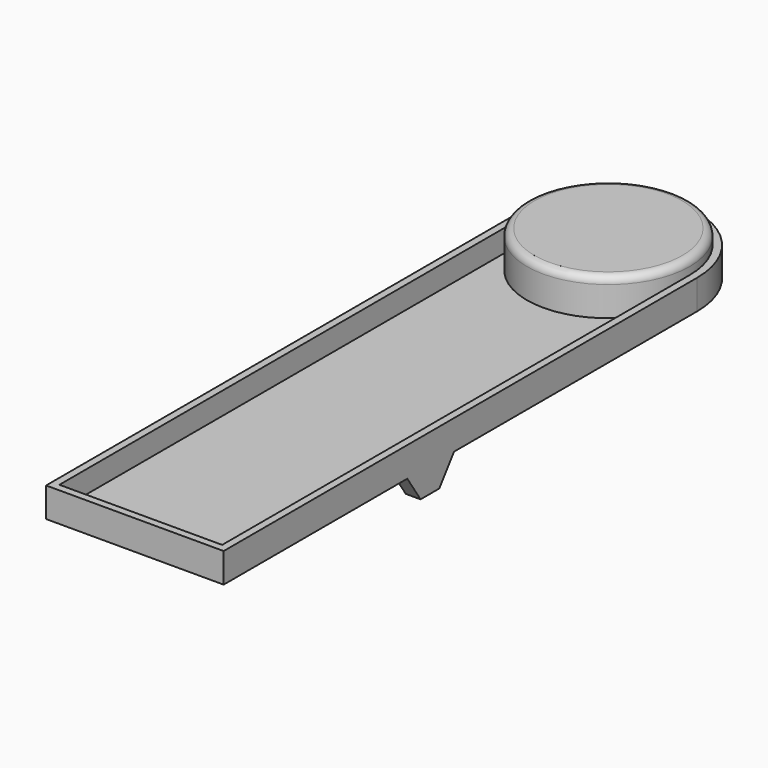
from build123d import *

# Parameters (mm, degrees)
F1_DEPTH = 50.8
F2_T     = -12.7
F3_R     = 139.7
F4_DEPTH = 63.5
F7_DEPTH = 25.4


# Not quite as in the source:
# - a fillet or chamfer that OpenCascade refuses, or shapes differently, is made with other operations: its cross-section is extruded or revolved along the edge and cut away or added


with BuildPart() as f1:
    # F0 (on Top) → F1 (new body)
    with BuildSketch(Plane.XY):
        with BuildLine():
            Line((152.4, -1016), (152.4, 0))
            ThreePointArc((152.4, 0), (0, -152.4), (-152.4, 0))
            Line((-152.4, 0), (-152.4, -1016))
            Line((-152.4, -1016), (152.4, -1016))
        make_face()
        with BuildLine():
            ThreePointArc((-152.4, 0), (0, -152.4), (152.4, 0))
            Line((152.4, 0), (-152.4, 0))
        make_face()
        with BuildLine():
            Line((-152.4, 0), (152.4, 0))
            ThreePointArc((152.4, 0), (0, 152.4), (-152.4, 0))
        make_face()
    extrude(amount=F1_DEPTH)

    # F2
    f2_openings = [f1.faces().sort_by_distance(p)[0] for p in [
        (0, -447.64327, 50.8),
    ]]
    offset(amount=F2_T, openings=f2_openings)

    # F3 (on face) → F4 (join)
    with BuildSketch(Plane.XY.offset(12.7)):
        Circle(F3_R)
        with BuildLine():
            ThreePointArc((-139.7, 0), (0, -139.7), (139.7, 0))
            ThreePointArc((139.7, 0), (0, 139.7), (-139.7, 0))
        make_face()
    extrude(amount=F4_DEPTH)

    # F5: fillet of radius 12.7 on 1 edges, made by hand

    # F5_s1 → F5_t2 (revolve, cut)
    with BuildSketch(Plane.XZ):
        with BuildLine():
            ThreePointArc((-139.7, 63.5), (-135.9802561211, 72.4802561211), (-127, 76.2))
            Line((-127, 76.2), (-139.7, 76.2))
            Line((-139.7, 76.2), (-139.7, 63.5))
        make_face()
    revolve(axis=Axis((0, 0, 76.2), (0, 0, 1)), mode=Mode.SUBTRACT)

    # F6 (on face) → F7 (join)
    with BuildSketch(Plane(origin=(-152.4, 0, 0), x_dir=(0, -1, 0), z_dir=(-1, 0, 0))):
        Polygon((621.9508647919, 0), (521.6426849365, 0), (553.3189177513, -42.8551286459), (593.4422016144, -42.8551286459), align=None)
    extrude(amount=-F7_DEPTH)

    # F8: F1 across plane


with BuildPart() as f1_1:
    add(f1.part)
    add(f1.part.mirror(Plane.YZ))


solid = f1_1.part
